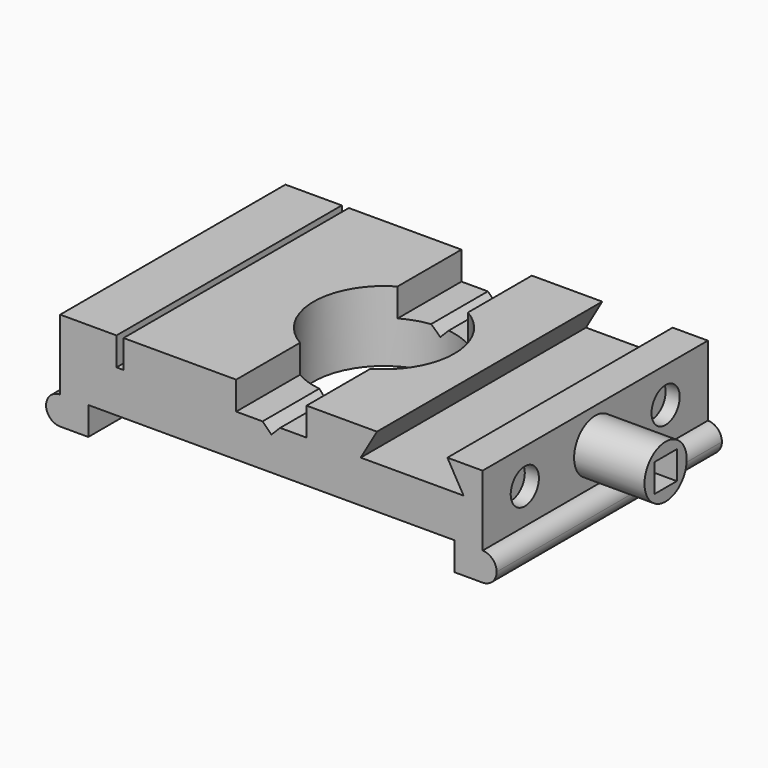
from build123d import *

# Parameters (mm, degrees)
F0_W      = 76.2
F0_H      = 50.8
F0_R      = 12.7
F1_DEPTH  = 12.7
F2_W      = 1.27
F2_H      = 50.8
F3_DEPTH  = 5.08
F5_DEPTH  = 50.801
F6_R      = 4.7625
F7_DEPTH  = 12.7
F8_W      = 5.08
F8_H      = 50.8
F9_DEPTH  = 5.08
F10_W     = 5.08
F10_H     = 5.08
F11_DEPTH = 12.7
F13_DEPTH = 50.8
F14_R     = 3.175
F15_DEPTH = 2.54
F17_DEPTH = 50.801


# Not quite as in the source:
# - a pattern or mirror of a feature is missing from the dataset's text; its kind, count and spacing are read off the source's solid


with BuildPart() as f1:
    # F0 (on Top) → F1 (new body)
    with BuildSketch(Plane.XY):
        Rectangle(F0_W, F0_H)
        Circle(F0_R, mode=Mode.SUBTRACT)
    extrude(amount=F1_DEPTH)

    # F2 (on face) → F3 (cut)
    with BuildSketch(Plane.XY.offset(12.7)):
        with Locations((-27.305, 0)):
            Rectangle(F2_W, F2_H)
        with BuildLine():
            Line((-6.35, -10.9985226281), (-6.35, -25.4))
            Line((-6.35, -25.4), (6.35, -25.4))
            Line((6.35, -25.4), (6.35, -10.9985226281))
            ThreePointArc((6.35, -10.9985226281), (0, -12.7), (-6.35, -10.9985226281))
        make_face()
        with BuildLine():
            Line((6.35, 25.4), (-6.35, 25.4))
            Line((-6.35, 25.4), (-6.35, 10.9985226281))
            ThreePointArc((-6.35, 10.9985226281), (0, 12.7), (6.35, 10.9985226281))
            Line((6.35, 10.9985226281), (6.35, 25.4))
        make_face()
    extrude(amount=-F3_DEPTH, mode=Mode.SUBTRACT)

    # F4 (on face) → F5 (cut, through all)
    with BuildSketch(Plane.XZ.offset(25.4)):
        Polygon((31.75, 12.7), (19.05, 12.7), (16.1170606325, 7.62), (34.6829393675, 7.62), align=None)
    extrude(amount=-F5_DEPTH, mode=Mode.SUBTRACT)

    # F6 (on face) → F7 (join)
    with BuildSketch(Plane.YZ.offset(38.1)):
        with Locations((0, 6.35)):
            Circle(F6_R)
    extrude(amount=F7_DEPTH)

    # F8 (on face) → F9 (join)
    with BuildSketch(Plane(origin=(0, 0, 0), x_dir=(1, 0, 0), z_dir=(0, 0, -1))):
        with Locations((-35.56, 0)):
            Rectangle(F8_W, F8_H)
        with Locations((35.56, 0)):
            Rectangle(F8_W, F8_H)
    extrude(amount=F9_DEPTH)

    # F10 (on face) → F11 (cut)
    with BuildSketch(Plane.YZ.offset(50.8)):
        with Locations((0, 6.35)):
            Rectangle(F10_W, F10_H)
    extrude(amount=-F11_DEPTH, mode=Mode.SUBTRACT)

    # F12 (on face) → F13 (join, through all)
    with BuildSketch(Plane.XZ.offset(25.4)):
        with BuildLine():
            ThreePointArc((38.1, -5.08), (39.8960512242, -4.3360512242), (40.64, -2.54))
            ThreePointArc((40.64, -2.54), (39.8960512242, -0.7439487758), (38.1, 0))
            Line((38.1, 0), (38.1, -5.08))
        make_face()
        with BuildLine():
            Line((38.1, -5.08), (38.1, 0))
            ThreePointArc((38.1, 0), (35.56, -2.54), (38.1, -5.08))
        make_face()
    f13 = extrude(amount=-F13_DEPTH)

    # F13_copies: F13 across plane
    add(f13.mirror(Plane(origin=(0, 0, 0), x_dir=(0, 0, -1), z_dir=(-1, 0, 0))))

    # F14 (on face) → F15 (cut)
    with BuildSketch(Plane.YZ.offset(38.1)):
        with Locations((-15.875, 6.35)):
            Circle(F14_R)
        with Locations((15.875, 6.35)):
            Circle(F14_R)
    extrude(amount=-F15_DEPTH, mode=Mode.SUBTRACT)

    # F16 (on face) → F17 (cut, through all)
    with BuildSketch(Plane.XZ.offset(25.4)):
        Polygon((-1.5875, 7.62), (0, 6.0325), (1.5875, 7.62), align=None)
    extrude(amount=-F17_DEPTH, mode=Mode.SUBTRACT)


solid = f1.part
